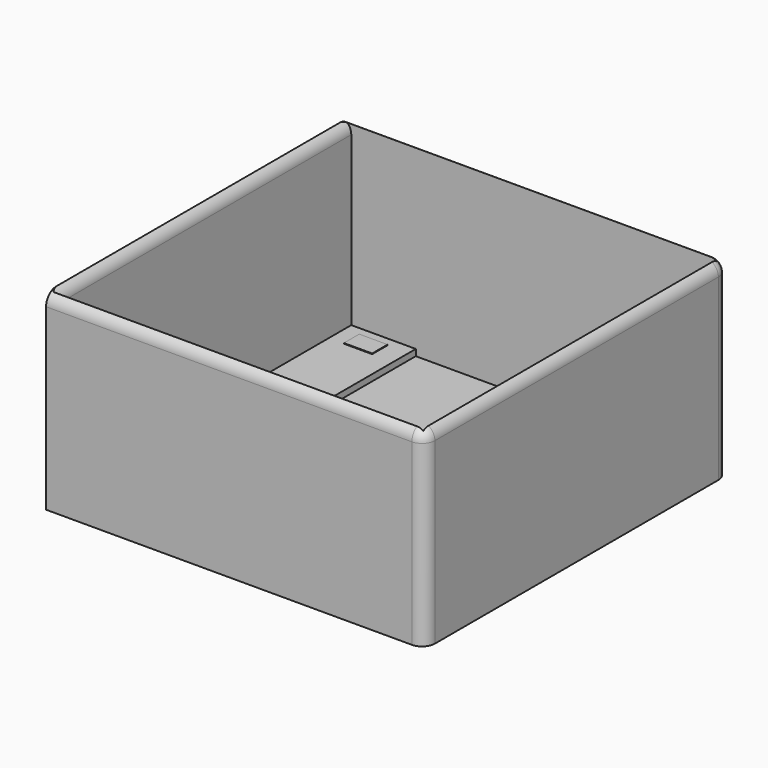
from build123d import *

# Parameters (mm, degrees)
F0_W        = 150.6382748485
F0_H        = 151.164598763
F1_DEPTH    = 76.2
F2_T        = -2.54
F3_T1_DEPTH = 176.0382748485
F4_T1_DEPTH = 158.784598763
F4_T3_DEPTH = 83.82
F4_T6_ANGLE = 89.9999999979
F5_T1_DEPTH = 158.2582748485
F5_T3_DEPTH = 83.82
F5_T6_ANGLE = 89.9999999979
F6_T4_DEPTH = 163.0016440191
F7_W        = 25.6696862793
F7_H        = 42.238175652
F8_DEPTH    = 2.54
F9_W        = 11.248614639
F9_H        = 7.6456852257
F10_DEPTH   = 0.254


# Not quite as in the source:
# - a fillet or chamfer that OpenCascade refuses, or shapes differently, is made with other operations: its cross-section is extruded or revolved along the edge and cut away or added


with BuildPart() as f1:
    # F0 (on Top) → F1 (new body)
    with BuildSketch(Plane.XY):
        with Locations((-0.1240856946, -0.0716410577)):
            Rectangle(F0_W, F0_H)
    extrude(amount=F1_DEPTH)

    # F2
    f2_openings = [f1.faces().sort_by_distance(p)[0] for p in [
        (-0.124086, -0.071641, 76.2),
    ]]
    offset(amount=F2_T, openings=f2_openings)

    # F3: fillet of radius 5.08 on 1 edges, made by hand

    # F3_s2 → F3_t1 (cut)
    with BuildSketch(Plane.YZ.offset(-88.1432231188)):
        with BuildLine():
            ThreePointArc((75.5106583238, 71.12), (74.0227607722, 74.7121024484), (70.4306583238, 76.2))
            Line((70.4306583238, 76.2), (75.5106583238, 76.2))
            Line((75.5106583238, 76.2), (75.5106583238, 71.12))
        make_face()
    extrude(amount=F3_T1_DEPTH, mode=Mode.SUBTRACT)

    # F4: fillet of radius 5.08 on 1 edges, made by hand

    # F4_s2 → F4_t1 (cut)
    with BuildSketch(Plane.XZ.offset(-70.4306583238)):
        with BuildLine():
            ThreePointArc((70.1150517297, 76.2), (73.7071541781, 74.7121024484), (75.1950517297, 71.12))
            Line((75.1950517297, 71.12), (75.1950517297, 76.2))
            Line((75.1950517297, 76.2), (70.1150517297, 76.2))
        make_face()
    extrude(amount=F4_T1_DEPTH, mode=Mode.SUBTRACT)

    # F4_s4 → F4_t3 (cut)
    with BuildSketch(Plane.XY.offset(-12.7)):
        with BuildLine():
            ThreePointArc((70.1150517297, 75.5106583238), (73.7071541781, 74.0227607722), (75.1950517297, 70.4306583238))
            Line((75.1950517297, 70.4306583238), (75.1950517297, 75.5106583238))
            Line((75.1950517297, 75.5106583238), (70.1150517297, 75.5106583238))
        make_face()
    extrude(amount=F4_T3_DEPTH, mode=Mode.SUBTRACT)

    # F4_s5 → F4_t6 (revolve, cut)
    with BuildSketch(Plane.XZ.offset(-70.4306583237)):
        with BuildLine():
            ThreePointArc((70.1150517297, 76.2), (73.7071541781, 74.7121024484), (75.1950517297, 71.12))
            Line((75.1950517297, 71.12), (75.1950517297, 76.2))
            Line((75.1950517297, 76.2), (70.1150517297, 76.2))
        make_face()
    revolve(axis=Axis((75.1950517297, 70.4306583237, 71.1199999999), (-1, 0, 0)), revolution_arc=F4_T6_ANGLE, mode=Mode.SUBTRACT)

    # F5: fillet of radius 5.08 on 1 edges, made by hand

    # F5_s2 → F5_t1 (cut)
    with BuildSketch(Plane.YZ.offset(-88.1432231188)):
        with BuildLine():
            ThreePointArc((-75.6539404392, 71.12), (-74.1660428877, 74.7121024484), (-70.5739404392, 76.2))
            Line((-70.5739404392, 76.2), (-75.6539404392, 76.2))
            Line((-75.6539404392, 76.2), (-75.6539404392, 71.12))
        make_face()
    extrude(amount=F5_T1_DEPTH, mode=Mode.SUBTRACT)

    # F5_s4 → F5_t3 (cut)
    with BuildSketch(Plane.XY.offset(-12.7)):
        with BuildLine():
            ThreePointArc((70.1150517297, -75.6539404392), (73.7071541781, -74.1660428877), (75.1950517297, -70.5739404392))
            Line((75.1950517297, -70.5739404392), (75.1950517297, -75.6539404392))
            Line((75.1950517297, -75.6539404392), (70.1150517297, -75.6539404392))
        make_face()
    extrude(amount=F5_T3_DEPTH, mode=Mode.SUBTRACT)

    # F5_s5 → F5_t6 (revolve, cut)
    with BuildSketch(Plane.YZ.offset(70.1150517296)):
        with BuildLine():
            ThreePointArc((-75.6539404392, 71.12), (-74.1660428877, 74.7121024484), (-70.5739404392, 76.2))
            Line((-70.5739404392, 76.2), (-75.6539404392, 76.2))
            Line((-75.6539404392, 76.2), (-75.6539404392, 71.12))
        make_face()
    revolve(axis=Axis((70.1150517296, -75.6539404392, 71.1199999999), (0, 1, 0)), revolution_arc=F5_T6_ANGLE, mode=Mode.SUBTRACT)

    # F6: fillet of radius 5.08 on 1 edges, made by hand


with BuildPart() as f6_tool2:
    # F6_s3 → F6_t4 (new body)
    with BuildSketch(Plane.XZ.offset(-81.4291809519)):
        with BuildLine():
            ThreePointArc((-75.4432231188, 76.2), (-73.5838140676, 74.3405909488), (-72.9032231188, 71.8005909488))
            Line((-72.9032231188, 71.8005909488), (-72.9032231188, 76.2))
            Line((-72.9032231188, 76.2), (-75.4432231188, 76.2))
        make_face()
    extrude(amount=F6_T4_DEPTH)

    split(bisect_by=Plane.XZ.offset(73.1139404392), keep=Keep.BOTTOM)

    split(bisect_by=Plane.XZ.offset(-72.9706583238), keep=Keep.TOP)


with BuildPart() as f1_1:
    add(f1.part)

    # F6_t1: cut F6_tool2
    add(f6_tool2.part, mode=Mode.SUBTRACT)

    # F7 (on face) → F8 (join)
    with BuildSketch(Plane.XY.offset(2.54)):
        with Locations((-60.0683799791, 51.8515704978)):
            Rectangle(F7_W, F7_H)
    extrude(amount=F8_DEPTH)

    # F9 (on face) → F10 (join)
    with BuildSketch(Plane.XY.offset(5.08)):
        with Locations((-61.2332168967, 65.5658598989)):
            Rectangle(F9_W, F9_H)
    extrude(amount=F10_DEPTH)


solid = f1_1.part
